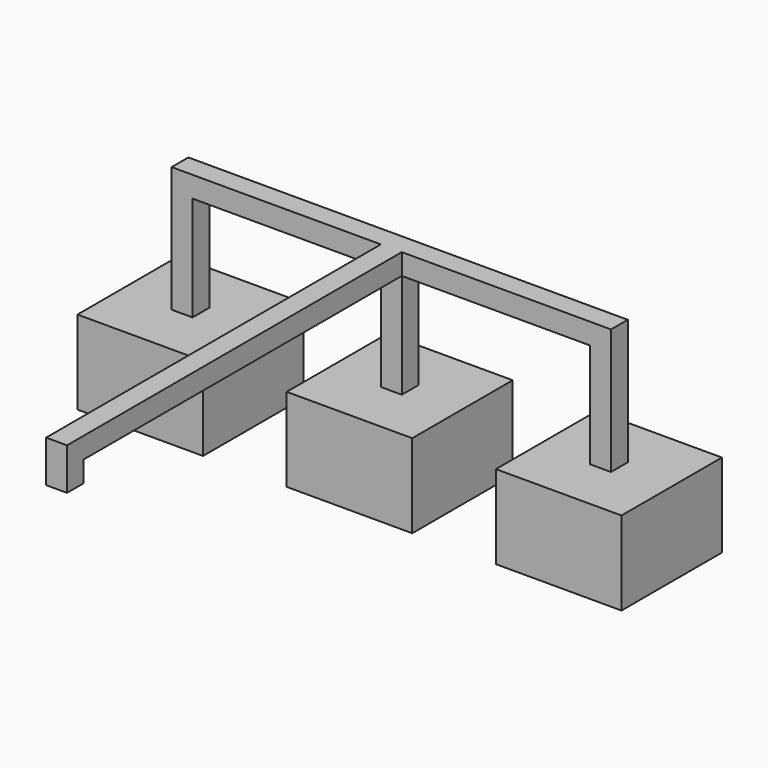
from build123d import *

# Parameters (mm, degrees)
F0_W      = 76.2
F0_H      = 76.2
F1_DEPTH  = 50.8
F3_W      = 12.7
F3_H      = 12.7
F5_DEPTH  = 76.2
F2_W      = 12.7
F2_H      = 12.7
F4_W      = 12.7
F4_H      = 12.7
F7_W      = 12.7
F7_H      = 12.7107013464
F8_DEPTH  = 114.3
F6_W      = 12.7
F6_H      = 12.7011348009
F9_W      = 12.7
F9_H      = 12.7
F10_DEPTH = 254
F11_W     = 12.7
F11_H     = 12.7
F12_DEPTH = 12.7


with BuildPart() as f1:
    # F0 (on Top) → F1 (new body)
    with BuildSketch(Plane.XY):
        with Locations((-127, 0)):
            Rectangle(F0_W, F0_H)
    extrude(amount=F1_DEPTH)


with BuildPart() as f1b:
    # F0 (on Top) → F1, piece 2 (new body)
    with BuildSketch(Plane.XY):
        Rectangle(F0_W, F0_H)
    extrude(amount=F1_DEPTH)


with BuildPart() as f1c:
    # F0 (on Top) → F1, piece 3 (new body)
    with BuildSketch(Plane.XY):
        with Locations((127, 0)):
            Rectangle(F0_W, F0_H)
    extrude(amount=F1_DEPTH)


with BuildPart() as f5:
    # F3 (on face) → F5 (new body)
    with BuildSketch(Plane.XY.offset(50.8)):
        with Locations((-127, 0)):
            Rectangle(F3_W, F3_H)
    extrude(amount=F5_DEPTH)



with BuildPart() as f5b:
    # F2 (on face) → F5, piece 2 (new body)
    with BuildSketch(Plane.XY.offset(50.8)):
        Rectangle(F2_W, F2_H)
    extrude(amount=F5_DEPTH)



with BuildPart() as f5c:
    # F4 (on face) → F5, piece 3 (new body)
    with BuildSketch(Plane.XY.offset(50.8)):
        with Locations((127, 0)):
            Rectangle(F4_W, F4_H)
    extrude(amount=F5_DEPTH)


with BuildPart() as f5b_1:
    add(f5b.part)

    add(f5c.part)  # F8 merges F5c
    # F7 (on face) → F8 (join)
    with BuildSketch(Plane.YZ.offset(6.35)):
        with Locations((0, 120.6446493268)):
            Rectangle(F7_W, F7_H)
    extrude(amount=F8_DEPTH)


with BuildPart() as f5_1:
    add(f5.part)

    add(f5b_1.part)  # F8#2 merges F5b
    # F6 (on face) → F8, piece 2 (join)
    with BuildSketch(Plane.YZ.offset(-120.65)):
        with Locations((0, 120.6494325995)):
            Rectangle(F6_W, F6_H)
    extrude(amount=F8_DEPTH)

    # F9 (on face) → F10 (join)
    with BuildSketch(Plane.XZ.offset(6.35)):
        with Locations((0, 120.65)):
            Rectangle(F9_W, F9_H)
    extrude(amount=F10_DEPTH)

    # F11 (on face) → F12 (join)
    with BuildSketch(Plane(origin=(0, 0, 114.3), x_dir=(1, 0, 0), z_dir=(0, 0, -1))):
        with Locations((0, 254)):
            Rectangle(F11_W, F11_H)
    extrude(amount=F12_DEPTH)


solid = Compound([f1.part, f1b.part, f1c.part, f5_1.part])
